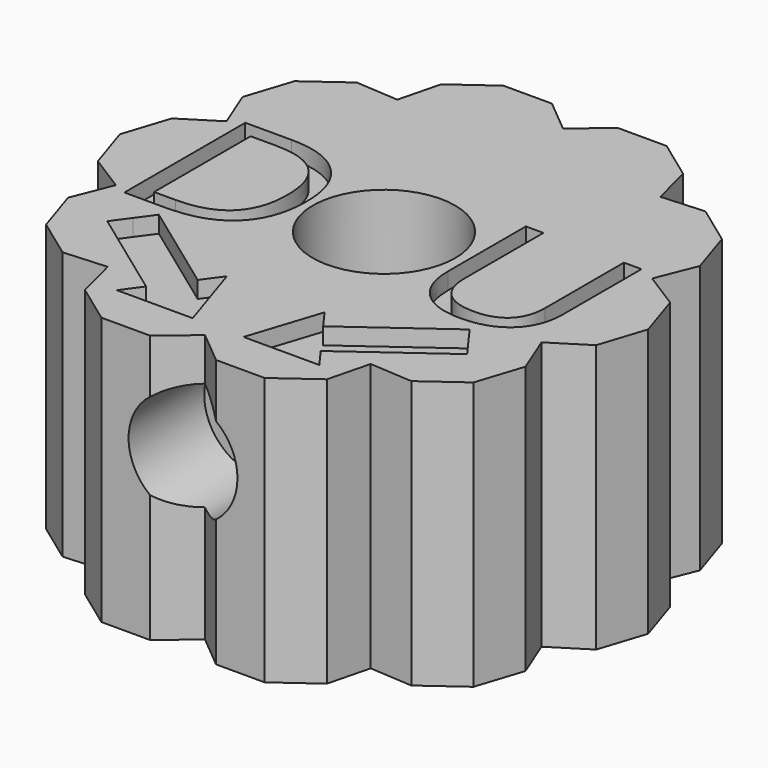
from build123d import *

# Parameters (mm, degrees)
F0_W           = 5.7
F0_H           = 2.7
F0_R           = 5.25
F0_R_2         = 4.25
F1_DEPTH       = 16
F2_DEPTH       = 7
F3_DEPTH       = 13.5
F5_D           = 3.3
F5_DEPTH       = 12
F5_START       = 1.6401413
F5_CBORE_D     = 6.5
F5_CBORE_DEPTH = 4
F5_TIP         = 0.9914200214
F6_TEXT_SIZE   = 12.6351453623
F7_DEPTH       = 1


# Not quite as in the source:
# - Text() gives the source's letters only with a copy of the font that has no kerning and outlines rounded to 1/6400 em; it was checked with that copy


with BuildPart() as f1:
    # F0 (on Top) → F1 (new body)
    with BuildSketch(Plane.XY):
        Polygon((14.8750668076, -2.7602714343), (15.7719333636, 0), (14.8750668076, 2.7602714343), (12.7059806301, 4.1284233667), (13.6566286812, 6.5102383969), (12.7597621253, 9.2705098312), (10.4117349984, 10.9764513958), (7.8527278898, 10.8083526939), (7.2218225704, 13.2940584354), (4.8737954435, 15), (1.9714743017, 15), (0, 13.3598586544), (-1.9714743017, 15), (-4.8737954435, 15), (-7.2218225704, 13.2940584354), (-7.8527278898, 10.8083526939), (-10.4117349984, 10.9764513958), (-12.7597621253, 9.2705098312), (-13.6566286812, 6.5102383969), (-12.7059806301, 4.1284233667), (-14.8750668076, 2.7602714343), (-15.7719333636, 0), (-14.8750668076, -2.7602714343), (-12.7059806301, -4.1284233667), (-13.6566286812, -6.5102383969), (-12.7597621253, -9.2705098312), (-10.4117349984, -10.9764513958), (-7.8527278898, -10.8083526939), (-7.2218225704, -13.2940584354), (-4.8737954435, -15), (-1.9714743017, -15), (0, -13.3598586544), (1.9714743017, -15), (4.8737954435, -15), (7.2218225704, -13.2940584354), (7.8527278898, -10.8083526939), (10.4117349984, -10.9764513958), (12.7597621253, -9.2705098312), (13.6566286812, -6.5102383969), (12.7059806301, -4.1284233667), align=None)
        with Locations((0, -7)):
            Rectangle(F0_W, F0_H, mode=Mode.SUBTRACT)
        Circle(F0_R, mode=Mode.SUBTRACT)
        Circle(F0_R)
        Circle(F0_R_2, mode=Mode.SUBTRACT)
        with Locations((0, -7)):
            Rectangle(F0_W, F0_H)
    extrude(amount=F1_DEPTH)

    # F0 (on Top) → F2 (cut)
    with BuildSketch(Plane.XY):
        Circle(F0_R)
        Circle(F0_R_2, mode=Mode.SUBTRACT)
    extrude(amount=F2_DEPTH, mode=Mode.SUBTRACT)

    # F0 (on Top) → F3 (cut)
    with BuildSketch(Plane.XY):
        with Locations((0, -7)):
            Rectangle(F0_W, F0_H)
    extrude(amount=F3_DEPTH, mode=Mode.SUBTRACT)

    # F5
    # its depths count from where the whole tool has entered the part; down to there all is cleared
    with Locations(Plane.XZ.offset(15).offset(-F5_START)):
        with Locations((0, 10.2)):
            CounterBoreHole(F5_D / 2, F5_CBORE_D / 2, F5_CBORE_DEPTH, depth=F5_DEPTH)
            with Locations((0, 0, -(F5_DEPTH + F5_TIP / 2))):  # 118° drill point
                Cone(0, F5_D / 2, F5_TIP, mode=Mode.SUBTRACT)

    # F6 (on face) → F7 (cut)
    with BuildSketch(Plane.XY.offset(16)):
        with Locations((-13.1704751402, -4.4632874342)):
            Text('D', F6_TEXT_SIZE, font='Open Sans', text_align=(TextAlign.LEFT, TextAlign.BOTTOM))
        with Locations((3.6761085503, -4.4632874342)):
            Text('U', F6_TEXT_SIZE, font='Open Sans', text_align=(TextAlign.LEFT, TextAlign.BOTTOM))
        Polygon((-10.0099493592, -6.2140125833), (-10.7427157859, -7.222579045), (-5.2122161414, -11.2407222379), (-6.0430788435, -12.3843066394), (-1.5172681764, -12.3843066394), align=None)
        Polygon((-9.2771829324, -5.2054461216), (-10.0099493592, -6.2140125833), (-1.5172681764, -12.3843066394), (-2.9158205858, -8.0800049129), (-3.7466832879, -9.2235893145), align=None)
        Polygon((10.0099493592, -6.2140125833), (9.2771829324, -5.2054461216), (3.7466832879, -9.2235893145), (2.9158205858, -8.0800049129), (1.5172681764, -12.3843066394), (6.0430788435, -12.3843066394), (5.2122161414, -11.2407222379), (10.7427157859, -7.222579045), align=None)
    extrude(amount=-F7_DEPTH, mode=Mode.SUBTRACT)


solid = f1.part
